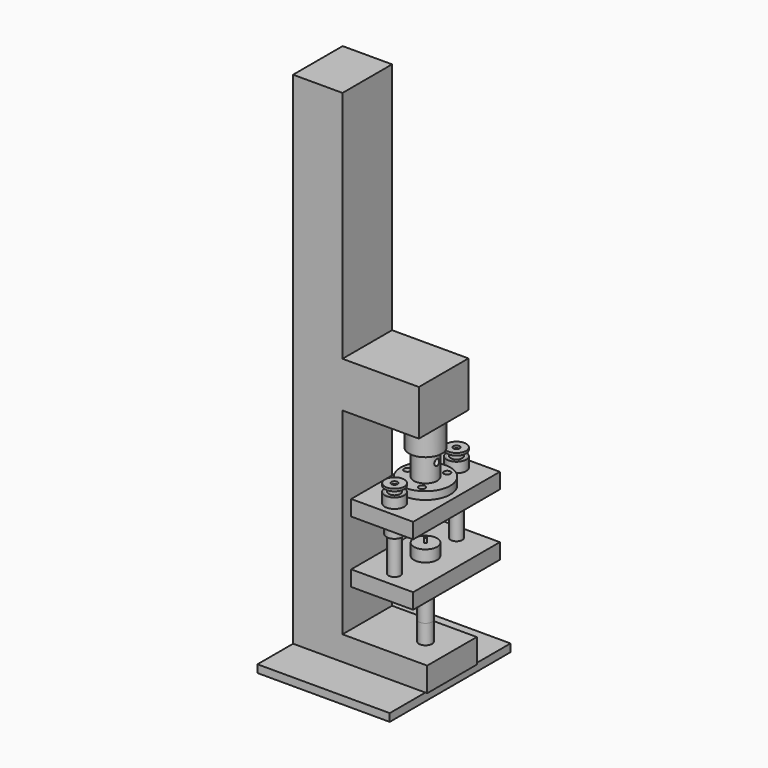
from build123d import *

# Parameters (mm, degrees)
F2_W           = 80
F2_H           = 140
F3_DEPTH       = 20
F5_W           = 80
F5_H           = 140
F6_DEPTH       = 20
F8_D           = 25
F9_D           = 15
F10_R          = 12.5
F10_R_2        = 10.5
F11_DEPTH      = 13
F11_DEPTH_BACK = 20
F12_R          = 7.5
F13_DEPTH      = 100
F13_DEPTH_BACK = 20
F14_SIZE2      = 0.8038475773
F14_SIZE       = 3
F16_D          = 5
F16_DEPTH      = 18
F16_TIP        = 1.5021515476
F17_R          = 12.5
F17_R_2        = 4
F18_DEPTH      = 3
F20_R          = 10.5
F20_R_2        = 7.5
F21_DEPTH      = 48
F25_R          = 10
F26_DEPTH      = 22
F27_R          = 4
F28_DEPTH      = 40.001
F28_DEPTH_BACK = 40.001
F30_D          = 8.5
F31_D          = 5
F32_R          = 15
F33_DEPTH      = 15
F35_D          = 5
F35_DEPTH      = 8
F35_TIP        = 1.5021515476
F36_R          = 15
F37_DEPTH      = 15
F38_D          = 6.8
F38_DEPTH      = 13
F38_TIP        = 2.0429261047
F39_D          = 5
F39_2_D        = 5
F40_R          = 1.5
F41_DEPTH      = 6
F43_DEPTH      = 40
F43_DEPTH_BACK = 40
F44_R          = 21.2062603524
F45_DEPTH      = 34
F46_R          = 8.372976597
F47_DEPTH      = 25
F48_W          = 170.8134700563
F48_H          = 194.9852970555
F49_DEPTH      = 10
F50_DEPTH      = 52.8


with BuildPart() as f3:
    # F2 (on Top) → F3 (new body)
    with BuildSketch(Plane.XY):
        Rectangle(F2_W, F2_H)
    extrude(amount=-F3_DEPTH)

    # F8 (through all)
    with Locations(Plane.XY):
        with Locations((0, -50), (0, 50)):
            Hole(F8_D / 2)

    # F38
    with Locations(Plane.XY):
        with Locations((11.75, 20.3515969889), (-23.5, 0), (11.75, -20.3515969889)):
            Hole(F38_D / 2, depth=F38_DEPTH)
            with Locations((0, 0, -(F38_DEPTH + F38_TIP / 2))):  # 118° drill point
                Cone(0, F38_D / 2, F38_TIP, mode=Mode.SUBTRACT)

    # F39 (through all)
    with Locations(Plane.XY):
        with Locations((0, 0)):
            Hole(F39_D / 2)


with BuildPart() as f6:
    # F5 (on offset) → F6 (new body)
    with BuildSketch(Plane(origin=(0, 0, -80), x_dir=(1, 0, 0), z_dir=(0, 0, -1))):
        Rectangle(F5_W, F5_H)
    extrude(amount=F6_DEPTH)

    # F9 (through all)
    with Locations(Plane.XY):
        with Locations((0, -50), (0, 50)):
            Hole(F9_D / 2)

    # F39#2 (through all)
    with Locations(Plane.XY):
        with Locations((0, 0)):
            Hole(F39_2_D / 2)


with BuildPart() as f11:
    # F10 (on Top) → F11 (new body, two sides)
    with BuildSketch(Plane.XY) as f11_sk:
        with Locations((0, -50)):
            Circle(F10_R)
        with Locations((0, -50)):
            Circle(F10_R_2, mode=Mode.SUBTRACT)
    extrude(amount=F11_DEPTH)
    extrude(f11_sk.sketch, amount=-F11_DEPTH_BACK)


with BuildPart() as f13:
    # F12 (on offset) → F13 (new body, two sides)
    with BuildSketch(Plane(origin=(0, 0, -80), x_dir=(1, 0, 0), z_dir=(0, 0, -1))) as f13_sk:
        with Locations((0, 50)):
            Circle(F12_R)
    extrude(amount=-F13_DEPTH)
    extrude(f13_sk.sketch, amount=F13_DEPTH_BACK)

    # F14
    f14_edges = [f13.edges().sort_by_distance(p)[0] for p in [
        (-7.5, -50, 20),
    ]]
    f14_side = f13.faces().sort_by_distance((-7.5, -50, -40))[0]
    chamfer(f14_edges, length=F14_SIZE, length2=F14_SIZE2, reference=f14_side)

    # F16
    with Locations(Plane.XY.offset(20)):
        with Locations((0, -50)):
            Hole(F16_D / 2, depth=F16_DEPTH)
            with Locations((0, 0, -(F16_DEPTH + F16_TIP / 2))):  # 118° drill point
                Cone(0, F16_D / 2, F16_TIP, mode=Mode.SUBTRACT)


with BuildPart() as f18:
    # F17 (on face) → F18 (new body)
    with BuildSketch(Plane.XY.offset(20)):
        with Locations((0, -50)):
            Circle(F17_R)
        with Locations((0, -50)):
            Circle(F17_R_2, mode=Mode.SUBTRACT)
    extrude(amount=F18_DEPTH)


with BuildPart() as f21:
    # F20 (on offset) → F21 (new body)
    with BuildSketch(Plane(origin=(0, 0, -35), x_dir=(1, 0, 0), z_dir=(0, 0, -1))):
        with Locations((0, 50)):
            Circle(F20_R)
        with Locations((0, 50)):
            Circle(F20_R_2, mode=Mode.SUBTRACT)
    extrude(amount=-F21_DEPTH)


with BuildPart() as f22_1:
    # F22: instance of F21
    add(f21.part.mirror(Plane.XZ))


with BuildPart() as f22_2:
    # F22: instance of F11
    add(f11.part.mirror(Plane.XZ))


with BuildPart() as f22_3:
    # F22: instance of F13
    add(f13.part.mirror(Plane.XZ))


with BuildPart() as f22_4:
    # F22: instance of F18
    add(f18.part.mirror(Plane.XZ))


with BuildPart() as f24:
    # F23 (on Right) → F24 (revolve)
    with BuildSketch(Plane.YZ):
        Polygon((0, 40), (0, 0), (32, 0), (32, 10), (15, 10), (15, 40), align=None)
    revolve(axis=Axis((0, 0, 35.5085860893), (0, 0, 1)))

    # F25 (on face) → F26 (cut)
    with BuildSketch(Plane.XY.offset(40)):
        Circle(F25_R)
    extrude(amount=-F26_DEPTH, mode=Mode.SUBTRACT)

    # F27 (on Right) → F28 (cut, two sides)
    with BuildSketch(Plane.YZ) as f28_sk:
        with Locations((0, 31)):
            Circle(F27_R)
    extrude(amount=-F28_DEPTH, mode=Mode.SUBTRACT)
    extrude(f28_sk.sketch, amount=F28_DEPTH_BACK, mode=Mode.SUBTRACT)

    # F30 (through all)
    with Locations(Plane(origin=(0, 0, 0), x_dir=(1, 0, 0), z_dir=(0, 0, -1))):
        with Locations((11.75, -20.3515969889), (-23.5, 0), (11.75, 20.3515969889)):
            Hole(F30_D / 2)

    # F31 (through all)
    with Locations(Plane(origin=(0, 0, 0), x_dir=(1, 0, 0), z_dir=(0, 0, -1))):
        with Locations((0, 0)):
            Hole(F31_D / 2)


with BuildPart() as f33:
    # F32 (on offset) → F33 (new body)
    with BuildSketch(Plane(origin=(0, 0, -80), x_dir=(1, 0, 0), z_dir=(0, 0, -1))):
        Circle(F32_R)
    extrude(amount=-F33_DEPTH)

    # F35
    with Locations(Plane(origin=(0, 0, -80), x_dir=(1, 0, 0), z_dir=(0, 0, -1))):
        with Locations((0, 0)):
            Hole(F35_D / 2, depth=F35_DEPTH)
            with Locations((0, 0, -(F35_DEPTH + F35_TIP / 2))):  # 118° drill point
                Cone(0, F35_D / 2, F35_TIP, mode=Mode.SUBTRACT)


with BuildPart() as f37:
    # F36 (on face) → F37 (new body)
    with BuildSketch(Plane(origin=(0, 0, -20), x_dir=(1, 0, 0), z_dir=(0, 0, -1))):
        Circle(F36_R)
    extrude(amount=F37_DEPTH)


with BuildPart() as f41:
    # F40 (on face) → F41 (new body)
    with BuildSketch(Plane.XY.offset(-65)):
        Circle(F40_R)
    extrude(amount=F41_DEPTH)


with BuildPart() as f43:
    # F42 (on Front) → F43 (new body, two sides)
    with BuildSketch(Plane.XZ) as f43_sk:
        Polygon((-75.2206221223, -177.5446087122), (-75.2206221223, 76.9988000393), (23.4228949994, 76.9988000393), (23.4228949994, 135.7356309891), (-75.2206221223, 135.7356309891), (-75.2206221223, 437.9788935184), (-139.0305459499, 437.9788935184), (-139.0305459499, -208.9575380087), (34.1650284827, -208.9575380087), (34.1650284827, -177.5446087122), align=None)
    extrude(amount=F43_DEPTH)
    extrude(f43_sk.sketch, amount=-F43_DEPTH_BACK)

    # F44 (on face) → F45 (join)
    with BuildSketch(Plane(origin=(0, 0, 76.9988000393), x_dir=(1, 0, 0), z_dir=(0, 0, -1))):
        Circle(F44_R)
    extrude(amount=F45_DEPTH)

    # F46 (on face) → F47 (join)
    with BuildSketch(Plane.XY.offset(-177.5446087122)):
        Circle(F46_R)
    extrude(amount=F47_DEPTH)

    # F48 (on face) → F49 (join)
    with BuildSketch(Plane(origin=(0, 0, -208.9575380087), x_dir=(1, 0, 0), z_dir=(0, 0, -1))):
        with Locations((-53.6238109218, 0)):
            Rectangle(F48_W, F48_H)
    extrude(amount=F49_DEPTH)


with BuildPart() as f50:
    # F50 (new): a face of the model
    f50_faces = [f43.part.faces().sort_by_distance(p)[0] for p in [
        (0, 0, -152.5446087122),
    ]]
    extrude(f50_faces, amount=F50_DEPTH)


solid = Compound([f3.part, f6.part, f11.part, f13.part, f18.part, f21.part, f22_1.part, f22_2.part, f22_3.part, f22_4.part, f24.part, f33.part, f37.part, f41.part, f43.part, f50.part])
